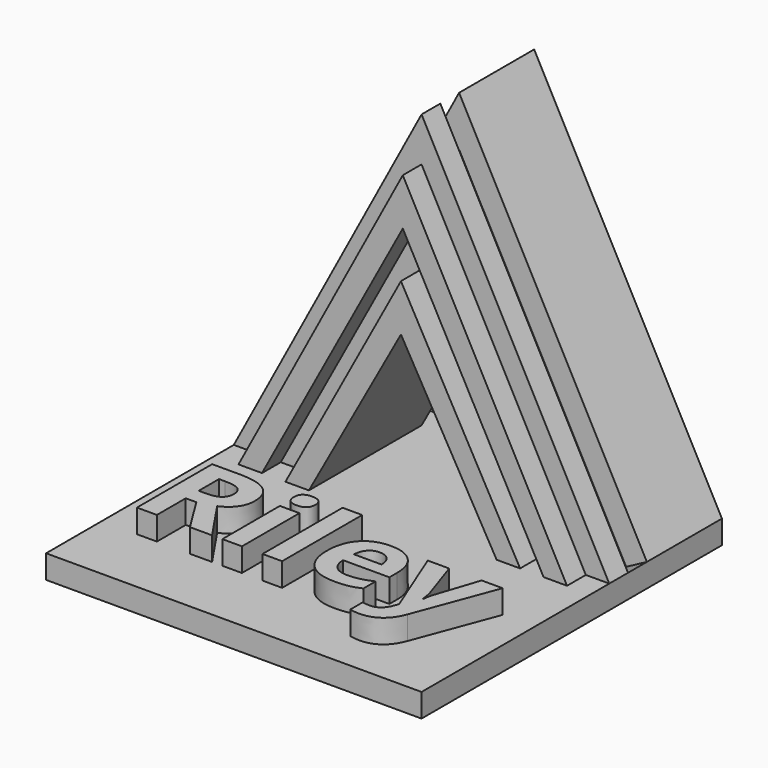
from build123d import *

# Parameters (mm, degrees)
F0_W          = 50.8
F0_H          = 50.8
F1_DEPTH      = 50.8
F2_W          = 50.8
F2_H          = 47.625
F3_DEPTH      = 31.75
F5_DEPTH      = 19.05
F8_DEPTH      = 3.175
F10_DEPTH     = 3.175
F12_DEPTH     = 22.225
F13_W         = 3.175
F13_H         = 53.975
F14_DEPTH     = 3.175
F15_W         = 3.175
F15_H         = 50.1517708333
F16_DEPTH     = 3.175
F18_DEPTH     = 3.175
F19_TEXT_SIZE = 17.8156312625
F20_DEPTH     = 3.175


# Not quite as in the source:
# - Text() gives the source's letters only with a copy of the font that has no kerning and outlines rounded to 1/6400 em; it was checked with that copy


with BuildPart() as f1:
    # F0 (on Front) → F1 (new body)
    with BuildSketch(Plane.XZ):
        with Locations((25.4, 25.4)):
            Rectangle(F0_W, F0_H)
    extrude(amount=F1_DEPTH)

    # F2 (on face) → F3 (cut)
    with BuildSketch(Plane.XZ.offset(50.8)):
        with Locations((25.4, 26.9875)):
            Rectangle(F2_W, F2_H)
    extrude(amount=-F3_DEPTH, mode=Mode.SUBTRACT)

    # F4 (on face) → F5 (cut)
    with BuildSketch(Plane.XZ.offset(19.05)):
        Polygon((0, 50.8), (0, 3.175), (25.4, 50.8), align=None)
        Polygon((50.8, 50.8), (25.4, 50.8), (50.8, 3.175), align=None)
    extrude(amount=-F5_DEPTH, mode=Mode.SUBTRACT)

    # F7 (on face) → F8 (join)
    with BuildSketch(Plane.XZ.offset(19.05)):
        Polygon((3.175, 3.175), (6.35, 3.175), (25.4000002316, 38.496875), (44.45, 3.175), (47.625, 3.175), (25.4, 44.846875), align=None)
    extrude(amount=F8_DEPTH)

    # F9 (on face) → F10 (join)
    with BuildSketch(Plane.XZ.offset(22.225)):
        Polygon((25.1528755332, 32.1516855321), (9.525, 3.175), (41.275, 3.175), align=None)
    extrude(amount=-F10_DEPTH)

    # F11 (on face) → F12 (cut)
    with BuildSketch(Plane.XZ.offset(22.225)):
        Polygon((25.1528755332, 25.8016855321), (12.7, 3.175), (38.1, 3.175), align=None)
    extrude(amount=-F12_DEPTH, mode=Mode.SUBTRACT)

    # F13 (on face) → F14 (cut)
    with BuildSketch(Plane(origin=(-1.3183391003, 0, 0.7031141869), x_dir=(0, -1, 0), z_dir=(-0.8823529412, 0, 0.4705882353))):
        with Locations((14.2875, 29.7889705882)):
            Rectangle(F13_W, F13_H)
    extrude(amount=-F14_DEPTH, mode=Mode.SUBTRACT)

    # F15 (on face) → F16 (cut)
    with BuildSketch(Plane(origin=(40.8685121107, 0, 21.7965397924), x_dir=(0, 1, 0), z_dir=(0.8823529412, 0, 0.4705882353))):
        with Locations((-14.2875, 3.971473652)):
            Rectangle(F15_W, F15_H)
    extrude(amount=-F16_DEPTH, mode=Mode.SUBTRACT)

    # F17 (on face) → F18 (cut)
    with BuildSketch(Plane(origin=(0, 0, 0), x_dir=(-1, 0, 0), z_dir=(0, 1, 0))):
        Polygon((-25.1528755332, 31.3503868479), (-41.275, 3.175), (-38.1, 3.175), (-25.1528755332, 25.8016855321), (-12.7, 3.175), (-9.525, 3.175), align=None)
    extrude(amount=-F18_DEPTH, mode=Mode.SUBTRACT)

    # F19 (on face) → F20 (join)
    with BuildSketch(Plane.XY.offset(3.175)):
        with Locations((3.175, -41.402254509)):
            Text('Riley', F19_TEXT_SIZE, font='Open Sans', font_style=FontStyle.BOLD, text_align=(TextAlign.LEFT, TextAlign.BOTTOM))
    extrude(amount=F20_DEPTH)


solid = f1.part
